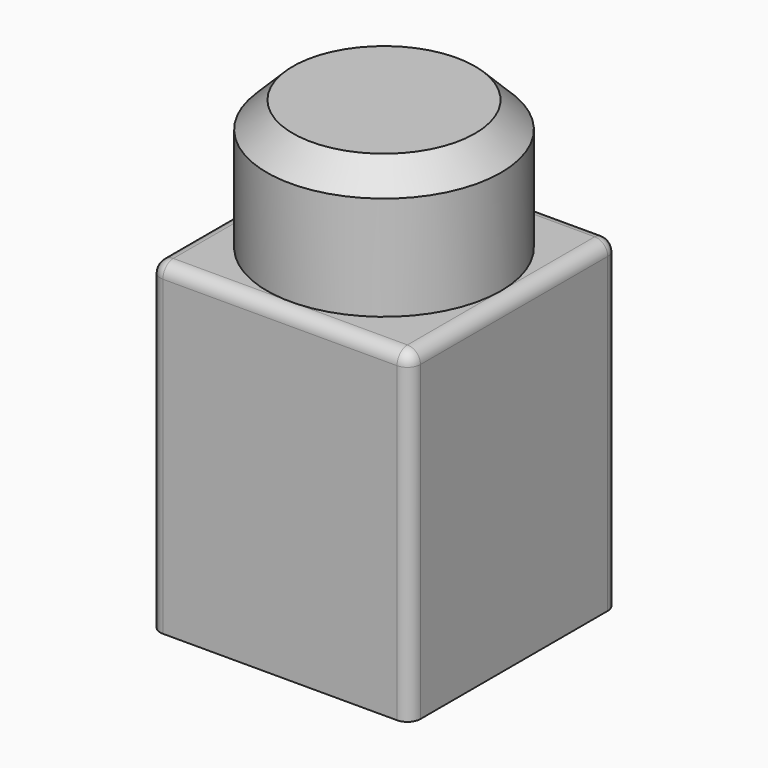
from build123d import *

# Parameters (mm, degrees)
F0_W     = 25.4
F0_H     = 25.4
F1_DEPTH = 31.75
F2_R     = 11.43
F3_DEPTH = 12.7
F4_SIZE  = 2.54
F5_R     = 1.27
F6_R     = 1.26999
F7_R     = 11.43
F8_DEPTH = 12.7


# Not quite as in the source:
# - a fillet or chamfer is up to 0.001 mm smaller than in the source, because OpenCascade refuses the exact size


with BuildPart() as f1:
    # F0 (on Top) → F1 (new body)
    with BuildSketch(Plane.XY):
        Rectangle(F0_W, F0_H)
    extrude(amount=F1_DEPTH)

    # F2 (on face) → F3 (join)
    with BuildSketch(Plane.XY.offset(31.75)):
        Circle(F2_R)
    extrude(amount=F3_DEPTH)

    # F4
    f4_edges = [f1.edges().sort_by_distance(p)[0] for p in [
        (-11.43, 0, 44.45),
    ]]
    chamfer(f4_edges, length=F4_SIZE)

    # F5
    f5_edges = [f1.edges().sort_by_distance(p)[0] for p in [
        (-12.7, -12.7, 15.875),
        (12.7, -12.7, 15.875),
        (-12.7, 12.7, 15.875),
        (12.7, 12.7, 15.875),
    ]]
    fillet(f5_edges, radius=F5_R)

    # F6 (radius 1.27 in the source; OpenCascade refuses exactly that, so slightly less here)
    f6_edges = [f1.edges().sort_by_distance(p)[0] for p in [
        (0, -12.7, 31.75),
        (12.7, 0, 31.75),
        (0, 12.7, 31.75),
        (-12.7, 0, 31.75),
    ]]
    fillet(f6_edges, radius=F6_R)

    # F7 (on face) → F8 (cut)
    with BuildSketch(Plane(origin=(0, 0, 0), x_dir=(1, 0, 0), z_dir=(0, 0, -1))):
        Circle(F7_R)
    extrude(amount=-F8_DEPTH, mode=Mode.SUBTRACT)


solid = f1.part
